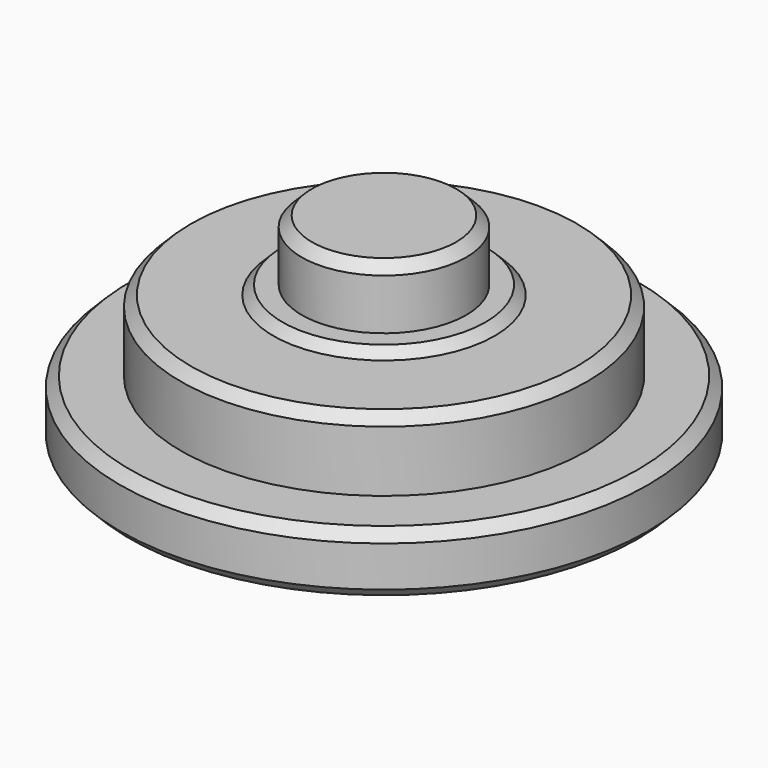
from build123d import *


# Not quite as in the source:
# - a fillet or chamfer that OpenCascade refuses, or shapes differently, is made with other operations: its cross-section is extruded or revolved along the edge and cut away or added


with BuildPart() as f1:
    # F0 (on Front) → F1 (revolve)
    with BuildSketch(Plane.XZ):
        Polygon((0, 9.95), (0, 0), (13, 0), (13, 3), (10, 3), (10, 6.5), (5.5, 6.5), (5.5, 6.95), (4.05, 6.95), (4.05, 9.95), align=None)
    revolve(axis=Axis((0, 0, 4.975), (0, 0, -1)))

    # F2: chamfer of 0.5 on 5 edges, made by hand

    # F2_s1 → F2_t2 (revolve, cut)
    with BuildSketch(Plane.XZ):
        Polygon((12.5, 0), (13, 0.5), (13, 0), align=None)
    revolve(axis=Axis((0, 0, 0), (0, 0, -1)), mode=Mode.SUBTRACT)

    # F2_s3 → F2_t4 (revolve, cut)
    with BuildSketch(Plane.XZ):
        Polygon((13, 2.5), (12.5, 3), (13, 3), align=None)
    revolve(axis=Axis((0, 0, 3), (0, 0, -1)), mode=Mode.SUBTRACT)

    # F2_s5 → F2_t6 (revolve, cut)
    with BuildSketch(Plane.XZ):
        Polygon((10, 6), (9.5, 6.5), (10, 6.5), align=None)
    revolve(axis=Axis((0, 0, 6.5), (0, 0, -1)), mode=Mode.SUBTRACT)


with BuildPart() as f2_tool8:
    # F2_s9 → F2_t10 (revolve)
    with BuildSketch(Plane.XZ):
        Polygon((5.5, 6.45), (5, 6.95), (5.5, 6.95), align=None)
    revolve(axis=Axis((0, 0, 6.95), (0, 0, -1)))

    split(bisect_by=Plane.XY.offset(6.5), keep=Keep.TOP)


with BuildPart() as f1_1:
    add(f1.part)

    # F2_t7: cut F2_tool8
    add(f2_tool8.part, mode=Mode.SUBTRACT)

    # F2_s12 → F2_t13 (revolve, cut)
    with BuildSketch(Plane.XZ):
        Polygon((4.05, 9.45), (3.55, 9.95), (4.05, 9.95), align=None)
    revolve(axis=Axis((0, 0, 9.95), (0, 0, -1)), mode=Mode.SUBTRACT)


solid = f1_1.part
